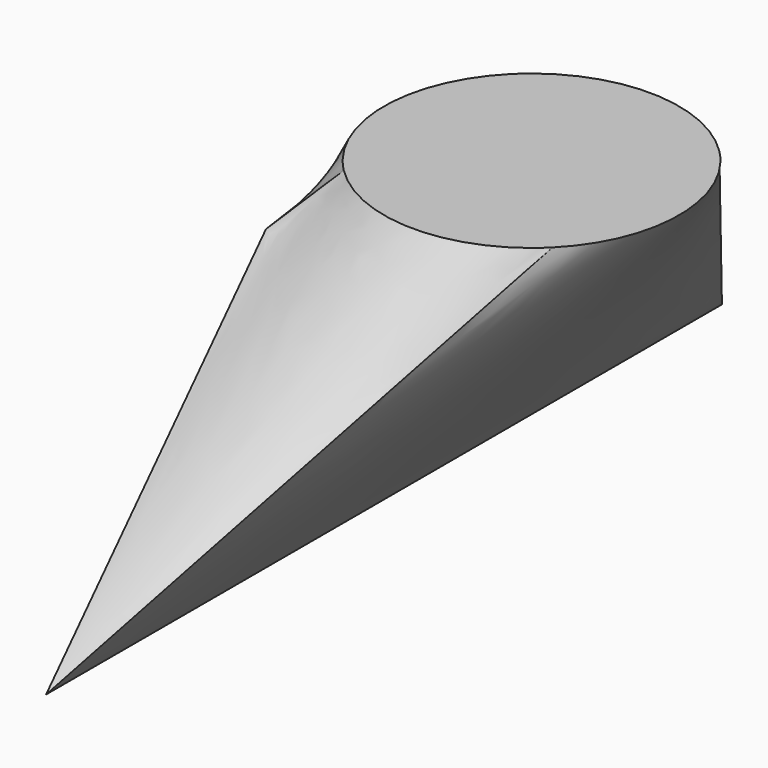
from build123d import *


# Not quite as in the source:
# - the arcs of a loft's sections are written as splines that run evenly, so that the points pair up as in the source's solid


with BuildPart() as f3:
    # F0 (on Top) → F3 section 0
    with BuildSketch(Plane.XY):
        with BuildLine():
            add(Edge.make_bspline(
                [(-7.0710678119, 7.0710678119), (-7.996668424, 6.1454671997), (-8.7378638835, 5.0361898037), (-9.7397267667, 2.6174788436), (-10, 1.308996939), (-10, -1.308996939), (-9.7397267667, -2.6174788436), (-8.7378638835, -5.0361898037), (-7.996668424, -6.1454671997), (-7.0710678119, -7.0710678119)],
                knots=[0, 0, 0, 0, 0.25, 0.25, 0.5, 0.5, 0.75, 0.75, 1, 1, 1, 1], degree=3))
            add(Edge.make_bspline(
                [(-7.0710678119, -7.0710678119), (-6.1454671997, -7.996668424), (-5.0361898037, -8.7378638835), (-2.6174788436, -9.7397267667), (-1.308996939, -10), (1.308996939, -10), (2.6174788436, -9.7397267667), (5.0361898037, -8.7378638835), (6.1454671997, -7.996668424), (7.0710678119, -7.0710678119)],
                knots=[0, 0, 0, 0, 0.25, 0.25, 0.5, 0.5, 0.75, 0.75, 1, 1, 1, 1], degree=3))
            add(Edge.make_bspline(
                [(7.0710678119, -7.0710678119), (7.996668424, -6.1454671997), (8.7378638835, -5.0361898037), (9.7397267667, -2.6174788436), (10, -1.308996939), (10, 1.308996939), (9.7397267667, 2.6174788436), (8.7378638835, 5.0361898037), (7.996668424, 6.1454671997), (7.0710678119, 7.0710678119)],
                knots=[0, 0, 0, 0, 0.25, 0.25, 0.5, 0.5, 0.75, 0.75, 1, 1, 1, 1], degree=3))
            add(Edge.make_bspline(
                [(7.0710678119, 7.0710678119), (6.1454671997, 7.996668424), (5.0361898037, 8.7378638835), (2.6174788436, 9.7397267667), (1.308996939, 10), (-1.308996939, 10), (-2.6174788436, 9.7397267667), (-5.0361898037, 8.7378638835), (-6.1454671997, 7.996668424), (-7.0710678119, 7.0710678119)],
                knots=[0, 0, 0, 0, 0.25, 0.25, 0.5, 0.5, 0.75, 0.75, 1, 1, 1, 1], degree=3))
        make_face()
    # F2 (on plane+point) → F3 section 1
    with BuildSketch(Plane.YZ.offset(-10)):
        Polygon((10, -3.2663967892), (-10, -3.2663967892), (-28.6285039037, -23.4635509551), (28.6285039037, -23.4635509551), align=None)
    loft(ruled=True)


solid = f3.part
